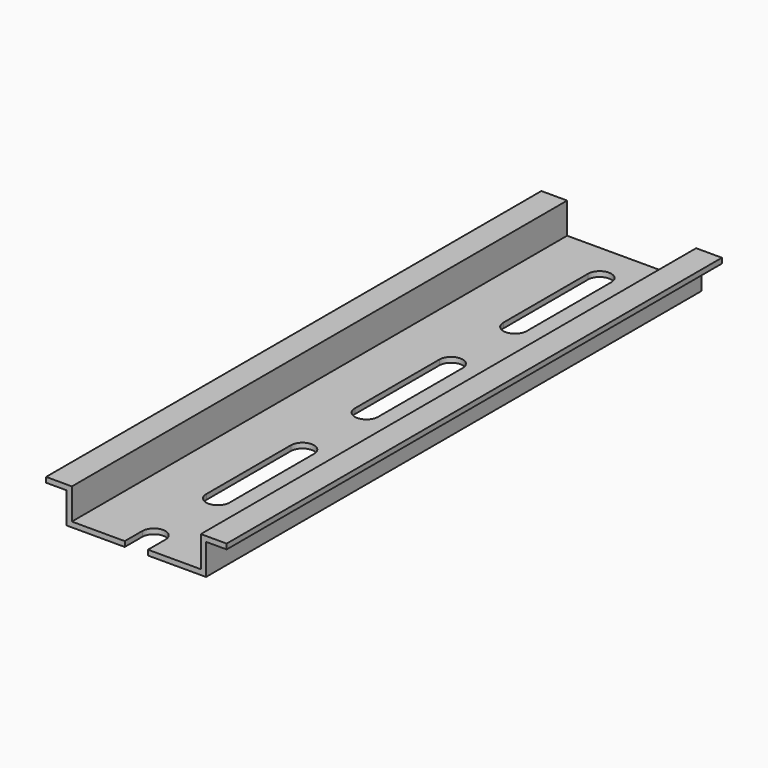
from build123d import *

# Parameters (mm, degrees)
F1_DEPTH = 120
F3_DEPTH = 1.001


# Not quite as in the source:
# - a feature names something its author has since deleted; it is built from what else it names


with BuildPart() as f1:
    # F0 (on Front) → F1 (new body)
    with BuildSketch(Plane.XZ):
        Polygon((-17.5, 6), (-17.5, 5), (-13.5, 5), (-13.5, -1), (13.5, -1), (13.5, 5), (17.5, 5), (17.5, 6), (12.5, 6), (12.5, 0), (-12.5, 0), (-12.5, 6), align=None)
    extrude(amount=F1_DEPTH)

    # F2 (on face) → F3 (cut, through all)
    with BuildSketch(Plane.XY):
        with BuildLine():
            ThreePointArc((-2.25, -28.25), (0, -30.5), (2.25, -28.25))
            Line((2.25, -28.25), (2.25, -7.75))
            ThreePointArc((2.25, -7.75), (0, -5.5), (-2.25, -7.75))
            Line((-2.25, -7.75), (-2.25, -28.25))
        make_face()
        with BuildLine():
            Line((-2.25, -43.75), (-2.25, -64.25))
            ThreePointArc((-2.25, -64.25), (0, -66.5), (2.25, -64.25))
            Line((2.25, -64.25), (2.25, -43.75))
            ThreePointArc((2.25, -43.75), (0, -41.5), (-2.25, -43.75))
        make_face()
        with BuildLine():
            Line((-2.25, -79.75), (-2.25, -100.25))
            ThreePointArc((-2.25, -100.25), (0, -102.5), (2.25, -100.25))
            Line((2.25, -100.25), (2.25, -79.75))
            ThreePointArc((2.25, -79.75), (0, -77.5), (-2.25, -79.75))
        make_face()
        with BuildLine():
            Line((-2.25, -120), (-2.25, -136.25))
            ThreePointArc((-2.25, -136.25), (0, -138.5), (2.25, -136.25))
            Line((2.25, -136.25), (2.25, -120))
            Line((2.25, -120), (-2.25, -120))
        make_face()
        with BuildLine():
            Line((-2.25, -115.75), (-2.25, -120))
            Line((-2.25, -120), (2.25, -120))
            Line((2.25, -120), (2.25, -115.75))
            ThreePointArc((2.25, -115.75), (0, -113.5), (-2.25, -115.75))
        make_face()
    extrude(amount=-F3_DEPTH, mode=Mode.SUBTRACT)


solid = f1.part
